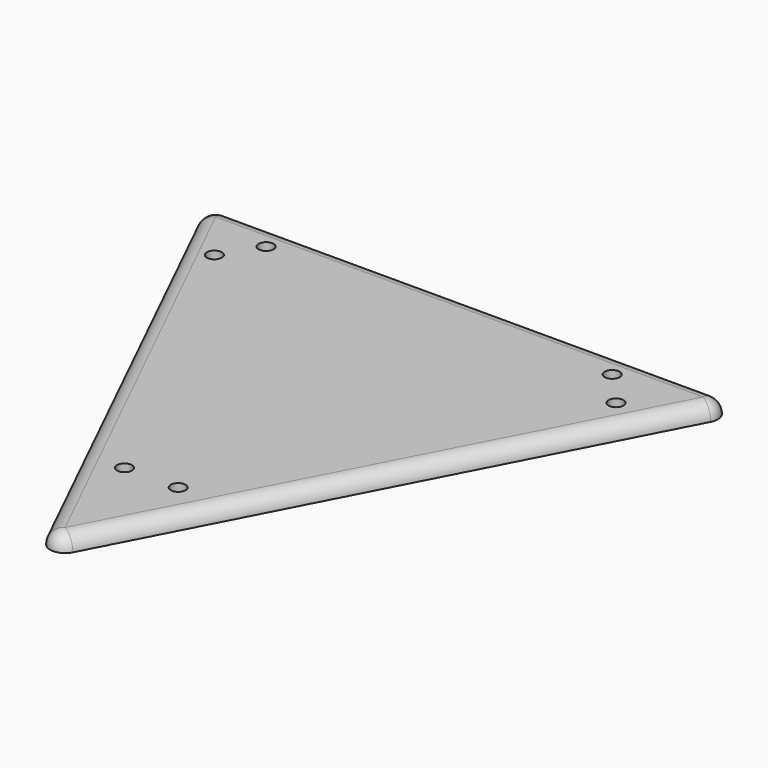
from build123d import *

# Parameters (mm, degrees)
F0_R     = 1.5933630383
F1_DEPTH = 3.175
F2_R     = 3.17499


# Not quite as in the source:
# - a fillet or chamfer is up to 0.001 mm smaller than in the source, because OpenCascade refuses the exact size


with BuildPart() as f1:
    # F0 (on Top) → F1 (new body)
    with BuildSketch(Plane.XY):
        Polygon((58.8864982128, 56.2052130699), (-55.4059632123, 56.2052130699), (0, -57.1772865951), align=None)
        with Locations((-5.6359637529, -27.1478164941)):
            Circle(F0_R, mode=Mode.SUBTRACT)
        with Locations((5.7859569788, -27.0903464407)):
            Circle(F0_R, mode=Mode.SUBTRACT)
        with Locations((-41.9265702367, 42.1965457499)):
            Circle(F0_R, mode=Mode.SUBTRACT)
        with Locations((-37.0861701667, 49.9411858618)):
            Circle(F0_R, mode=Mode.SUBTRACT)
        with Locations((43.6793863773, 42.3348434269)):
            Circle(F0_R, mode=Mode.SUBTRACT)
        with Locations((36.7645248771, 49.9411858618)):
            Circle(F0_R, mode=Mode.SUBTRACT)
    extrude(amount=F1_DEPTH)

    # F2 (radius 3.175 in the source; OpenCascade refuses exactly that, so slightly less here)
    f2_edges = [f1.edges().sort_by_distance(p)[0] for p in [
        (-27.702982, -0.486037, 3.175),
        (29.443249, -0.486037, 3.175),
        (1.740268, 56.205213, 3.175),
        (0, -57.177287, 1.5875),
        (-55.405963, 56.205213, 1.5875),
        (58.886498, 56.205213, 1.5875),
    ]]
    fillet(f2_edges, radius=F2_R)


solid = f1.part
